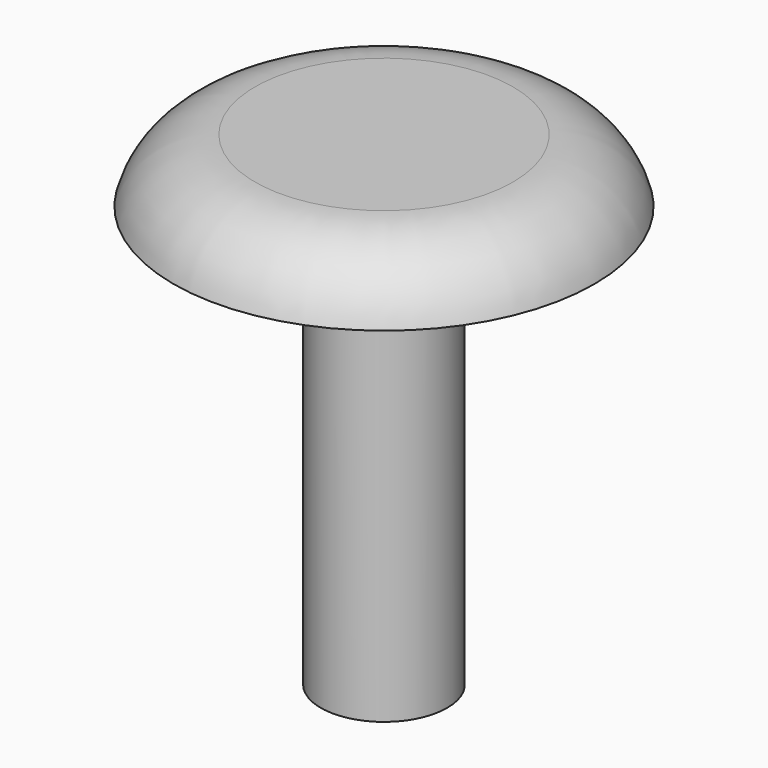
from build123d import *

# Parameters (mm, degrees)
F0_R     = 3.81
F1_DEPTH = 25.4
F2_R     = 6.35
F2_R_2   = 3.81
F3_DEPTH = 3.81
F2_R_3   = 12.7
F4_DEPTH = 3.81


# Not quite as in the source:
# - a fillet or chamfer that OpenCascade refuses, or shapes differently, is made with other operations: its cross-section is extruded or revolved along the edge and cut away or added


with BuildPart() as f1:
    # F0 (on Top) → F1 (new body)
    with BuildSketch(Plane.XY):
        Circle(F0_R)
    extrude(amount=F1_DEPTH)

    # F2 (on face) → F3 (join)
    with BuildSketch(Plane.XY.offset(25.4)):
        Circle(F2_R)
        Circle(F2_R_2, mode=Mode.SUBTRACT)
        Circle(F2_R_2)
    extrude(amount=F3_DEPTH)

    # F2 (on face) → F4 (join)
    with BuildSketch(Plane.XY.offset(25.4)):
        Circle(F2_R_3)
        Circle(F2_R, mode=Mode.SUBTRACT)
    extrude(amount=F4_DEPTH)

    # F5: fillet of radius 5.08 on 1 edges, made by hand

    # F5_s1 → F5_t2 (revolve, cut)
    with BuildSketch(Plane.XZ):
        with BuildLine():
            ThreePointArc((12.7, 25.4), (10.8921631237, 28.1460926284), (7.7813111503, 29.21))
            Line((7.7813111503, 29.21), (12.7, 29.21))
            Line((12.7, 29.21), (12.7, 25.4))
        make_face()
    revolve(axis=Axis((0, 0, 29.21), (0, 0, 1)), mode=Mode.SUBTRACT)


solid = f1.part
